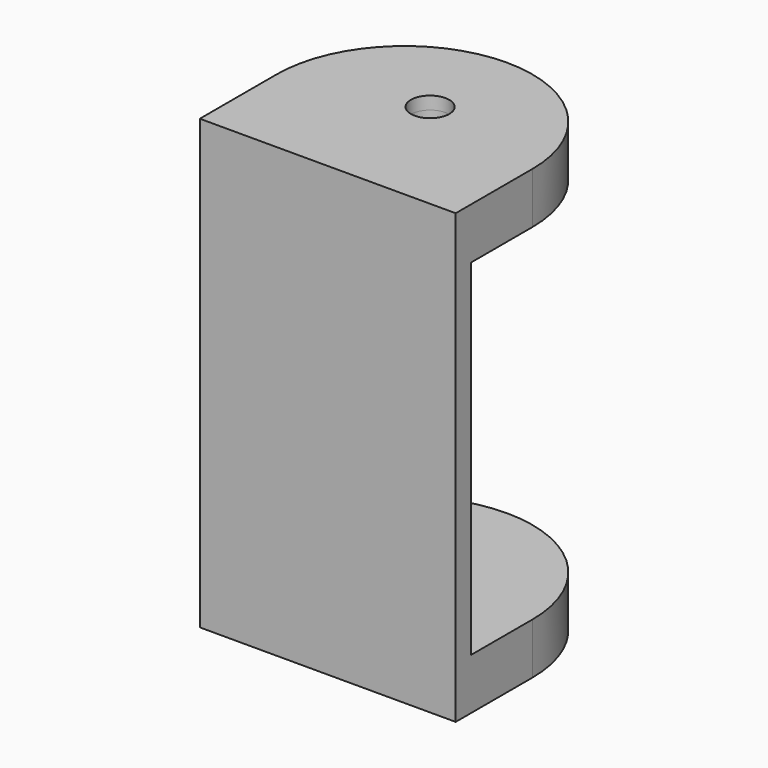
from build123d import *

# Parameters (mm, degrees)
F0_W     = 40
F0_H     = 35
F0_R     = 3
F1_DEPTH = 8
F2_DEPTH = 2
F3_W     = 40
F3_H     = 27
F4_DEPTH = 3
F5_R     = 20
F6_R     = 19.99999
F8_DEPTH = 2.001
F9_DEPTH = 2.001


# Not quite as in the source:
# - a fillet or chamfer is up to 0.001 mm smaller than in the source, because OpenCascade refuses the exact size


with BuildPart() as f1:
    # F0 (on Top) → F1 (new body)
    with BuildSketch(Plane.XY):
        Rectangle(F0_W, F0_H)
        with Locations((0, 2.5)):
            Circle(F0_R, mode=Mode.SUBTRACT)
    extrude(amount=F1_DEPTH)

    # F0 (on Top) → F2 (join)
    with BuildSketch(Plane.XY):
        with Locations((0, 2.5)):
            Circle(F0_R)
    extrude(amount=F2_DEPTH)

    # F3 (on face) → F4 (join)
    with BuildSketch(Plane.XZ.offset(17.5)):
        with Locations((0, 21.5)):
            Rectangle(F3_W, F3_H)
    extrude(amount=-F4_DEPTH)

    # F5
    f5_edges = [f1.edges().sort_by_distance(p)[0] for p in [
        (-20, 17.5, 4),
    ]]
    fillet(f5_edges, radius=F5_R)

    # F6 (radius 20 in the source; OpenCascade refuses exactly that, so slightly less here)
    f6_edges = [f1.edges().sort_by_distance(p)[0] for p in [
        (20, 17.5, 4),
    ]]
    fillet(f6_edges, radius=F6_R)

    # F7: F1 across face


with BuildPart() as f1_1:
    add(f1.part)
    add(f1.part.mirror(Plane(origin=(0, -16, 35), x_dir=(1, 0, 0), z_dir=(0, 0, 1))))

    # F8 (cut, through all): a face of the model
    f8_faces = [f1_1.faces().sort_by_distance(p)[0] for p in [
        (0, 2.5, 2),
    ]]
    extrude(f8_faces, amount=-F8_DEPTH, mode=Mode.SUBTRACT)

    # F9 (cut, through all): a face of the model
    f9_faces = [f1_1.faces().sort_by_distance(p)[0] for p in [
        (0, 2.5, 68),
    ]]
    extrude(f9_faces, amount=-F9_DEPTH, mode=Mode.SUBTRACT)


solid = f1_1.part
